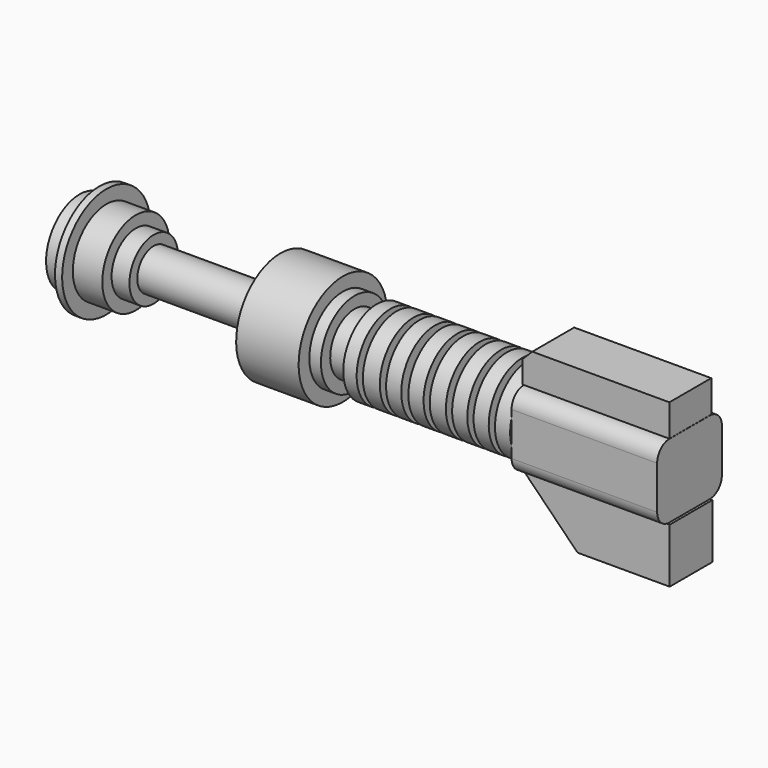
from build123d import *

# Parameters (mm, degrees)
F2_W      = 76.3007998466
F2_H      = 29.4303083792
F3_DEPTH  = 21.336
F4_DEPTH  = 21.082
F5_DEPTH  = 3.556
F6_DEPTH  = 5.588
F7_R      = 7.971733183
F8_R      = 7.9756
F9_R      = 7.9756
F10_R     = 7.9756
F11_W     = 76.9134834409
F11_H     = 16.80192817
F12_DEPTH = 13.716
F13_DEPTH = 13.716
F14_SIZE  = 5.08
F16_DEPTH = 13.97
F17_DEPTH = 13.97


# Not quite as in the source:
# - the program builds the solid bodies; features that only make, move or delete a surface that nothing else refers to are left out


with BuildPart() as f1:
    # F0 (on Front) → F1 (revolve)
    with BuildSketch(Plane.XZ):
        Polygon((-174.9170422554, 18.2400159538), (-174.9170422554, 0), (0, 0), (68.2831183076, 0), (68.2831183076, 12.1600115672), (68.2831183076, 18.2400159538), (60.3323429823, 18.2400159538), (60.3323429823, 12.1600115672), (57.0584982634, 12.1600115672), (57.0584982634, 18.2400159538), (49.1077229381, 18.2400159538), (49.1077229381, 12.1600115672), (45.8338782191, 12.1600115672), (45.8338782191, 18.2400159538), (37.8831028938, 18.2400159538), (37.8831028938, 12.1600115672), (34.609246999, 12.1600115672), (34.609246999, 18.2400159538), (26.1907801032, 18.2400159538), (26.1907801032, 12.1600115672), (22.9169353843, 12.1600115672), (22.9169353843, 18.2400159538), (14.966160059, 18.2400159538), (14.966160059, 12.1600115672), (11.2246191129, 12.1600115672), (11.2246191129, 18.2400159538), (3.2738437876, 18.2400159538), (3.2738437876, 12.1600115672), (0, 12.1600115672), (0, 18.2400159538), (-8.886160329, 18.2400159538), (-8.886160329, 12.1600115672), (-12.1600097045, 12.1600115672), (-12.1600097045, 18.2400159538), (-19.1753990948, 18.2400159538), (-19.1753990948, 12.1600115672), (-30.8677144349, 12.1600115672), (-30.8677144349, 18.2400159538), (-36.9477197528, 18.2400159538), (-36.9477197528, 25.2554044127), (-69.6861967444, 25.2554044127), (-69.6861967444, 12.1600115672), (-76.2338936329, 12.1600115672), (-76.2338936329, 7.0153931156), (-136.09854877, 7.0153931156), (-136.09854877, 12.1600115672), (-145.4523950815, 12.1600115672), (-145.4523950815, 18.2400159538), (-160.8862578869, 18.2400159538), (-160.8862578869, 25.2554044127), (-164.627790451, 25.2554044127), (-164.627790451, 18.2400159538), align=None)
    revolve(axis=Axis((-46.7692613602, 0, -3.7415372208), (1, 0, 0)))

    # F11 (on Front) → F12 (join)
    with BuildSketch(Plane.XZ):
        with Locations((106.6653989255, 23.5083936714)):
            Rectangle(F11_W, F11_H)
    extrude(amount=F12_DEPTH)

    # F13 (add): a face of the model
    f13_faces = [f1.faces().sort_by_distance(p)[0] for p in [
        (106.6723347987, 0, 23.5096275343),
    ]]
    extrude(f13_faces, amount=F13_DEPTH)

    # F14
    f14_edges = [f1.edges().sort_by_distance(p)[0] for p in [
        (68.208657, 0, 31.909358),
    ]]
    chamfer(f14_edges, length=F14_SIZE)


with BuildPart() as f3:
    # F2 (on Front) → F3 (new body)
    with BuildSketch(Plane.XZ):
        with Locations((106.6665202379, -3.4833862446)):
            Rectangle(F2_W, F2_H)
    extrude(amount=F3_DEPTH)

    # F4 (add): a face of the model
    f4_faces = [f3.faces().sort_by_distance(p)[0] for p in [
        (106.6665202379, 0, -3.4833862446),
    ]]
    extrude(f4_faces, amount=F4_DEPTH)

    # F5 (add): a face of the model
    f5_faces = [f3.faces().sort_by_distance(p)[0] for p in [
        (106.6665202379, -0.127, 11.231767945),
    ]]
    extrude(f5_faces, amount=F5_DEPTH)

    # F6 (add): a face of the model
    f6_faces = [f3.faces().sort_by_distance(p)[0] for p in [
        (106.6665202379, -0.127, -18.1985404342),
    ]]
    extrude(f6_faces, amount=F6_DEPTH)

    # F7
    f7_edges = [f3.edges().sort_by_distance(p)[0] for p in [
        (106.66652, -21.336, -23.78654),
    ]]
    fillet(f7_edges, radius=F7_R)

    # F8
    f8_edges = [f3.edges().sort_by_distance(p)[0] for p in [
        (106.66652, -21.336, 14.787768),
    ]]
    fillet(f8_edges, radius=F8_R)

    # F9
    f9_edges = [f3.edges().sort_by_distance(p)[0] for p in [
        (106.66652, 21.082, 14.787768),
    ]]
    fillet(f9_edges, radius=F9_R)

    # F10
    f10_edges = [f3.edges().sort_by_distance(p)[0] for p in [
        (106.66652, 21.082, -23.78654),
    ]]
    fillet(f10_edges, radius=F10_R)


with BuildPart() as f16:
    # F15 (on Front) → F16 (new body)
    with BuildSketch(Plane.XZ):
        Polygon((145.4702168703, -24.3446994573), (68.9654946327, -24.3446994573), (97.2078964114, -52.9445968568), (145.4702168703, -52.9445968568), align=None)
    extrude(amount=F16_DEPTH)

    # F17 (add): a face of the model
    f17_faces = [f16.faces().sort_by_distance(p)[0] for p in [
        (113.7457078297, 0, -37.565664242),
    ]]
    extrude(f17_faces, amount=F17_DEPTH)


solid = Compound([f1.part, f3.part, f16.part])
